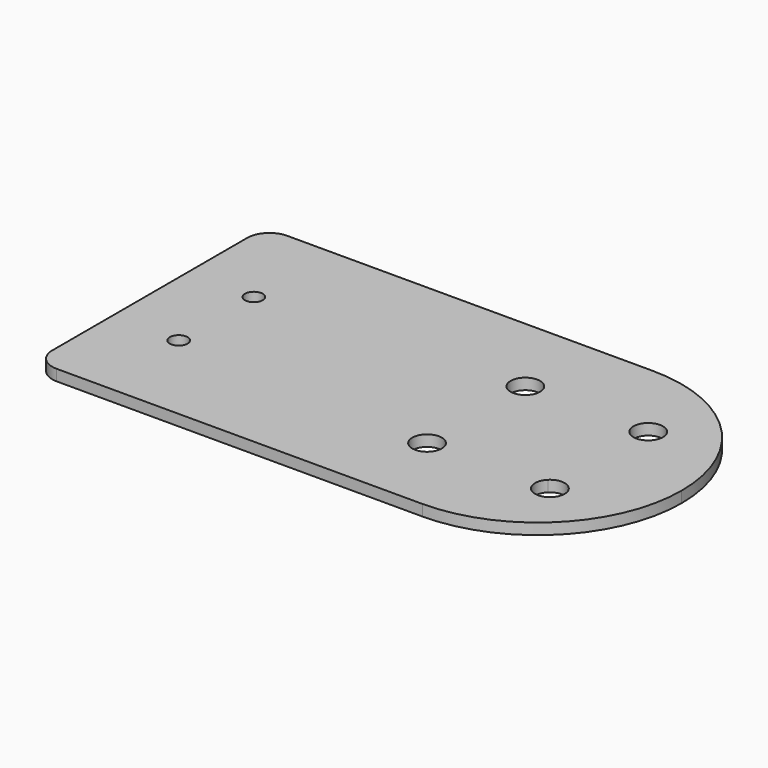
from build123d import *

# Parameters (mm, degrees)
F0_R     = 2.54
F1_DEPTH = 3.175


# Not quite as in the source:
# - a feature names something its author has since deleted; it is built from what else it names


with BuildPart() as f1:
    # F0 (on Top) → F1 (new body)
    with BuildSketch(Plane.XY):
        with BuildLine():
            ThreePointArc((-41.275, 0), (-29.1858323935, 29.1858323935), (0, 41.275))
            Line((0, 41.275), (-104.775, 41.275))
            ThreePointArc((-104.775, 41.275), (-109.2651280605, 39.4151280605), (-111.125, 34.925))
            Line((-111.125, 34.925), (-111.125, 0))
            Line((-111.125, 0), (-41.275, 0))
        make_face()
        with Locations((-92.075, 13.462)):
            Circle(F0_R, mode=Mode.SUBTRACT)
        with BuildLine():
            Line((-104.775, -41.275), (0, -41.275))
            ThreePointArc((0, -41.275), (-29.1858323935, -29.1858323935), (-41.275, 0))
            Line((-41.275, 0), (-111.125, 0))
            Line((-111.125, 0), (-111.125, -34.925))
            ThreePointArc((-111.125, -34.925), (-109.2651280605, -39.4151280605), (-104.775, -41.275))
        make_face()
        with Locations((-92.075, -13.462)):
            Circle(F0_R, mode=Mode.SUBTRACT)
        with BuildLine():
            Line((0, 2.8299858928), (0, 41.275))
            ThreePointArc((0, 41.275), (-29.1858323935, 29.1858323935), (-41.275, 0))
            Line((-41.275, 0), (0, 0))
            Line((0, 0), (0, 2.8299858928))
        make_face()
        with BuildLine():
            ThreePointArc((-13.3722019973, 17.6013019973), (-13.6941230664, 15.9828954935), (-14.610876709, 14.610876709))
            ThreePointArc((-14.610876709, 14.610876709), (-21.5084809282, 19.2197085011), (-13.3722019973, 17.6013019973))
        make_face(mode=Mode.SUBTRACT)
        with BuildLine():
            ThreePointArc((-41.275, 0), (-29.1858323935, -29.1858323935), (0, -41.275))
            Line((0, -41.275), (0, 0))
            Line((0, 0), (-41.275, 0))
        make_face()
        with BuildLine():
            ThreePointArc((-13.3722019973, -17.6013019973), (-21.5084809282, -19.2197085011), (-14.610876709, -14.610876709))
            ThreePointArc((-14.610876709, -14.610876709), (-13.6941230664, -15.9828954935), (-13.3722019973, -17.6013019973))
        make_face(mode=Mode.SUBTRACT)
        with BuildLine():
            ThreePointArc((0, -41.275), (29.1858323935, -29.1858323935), (41.275, 0))
            ThreePointArc((41.275, 0), (29.1858323935, 29.1858323935), (0, 41.275))
            Line((0, 41.275), (0, 2.8299858928))
            Line((0, 2.8299858928), (0, 0))
            Line((0, 0), (0, -41.275))
        make_face()
        with BuildLine():
            ThreePointArc((21.8304019973, -17.6013019973), (15.9828954935, -21.5084809282), (14.610876709, -14.610876709))
            ThreePointArc((14.610876709, -14.610876709), (19.2197085011, -13.6941230664), (21.8304019973, -17.6013019973))
        make_face(mode=Mode.SUBTRACT)
        with BuildLine():
            ThreePointArc((21.8304019973, 17.6013019973), (19.2197085011, 13.6941230664), (14.610876709, 14.610876709))
            ThreePointArc((14.610876709, 14.610876709), (15.9828954935, 21.5084809282), (21.8304019973, 17.6013019973))
        make_face(mode=Mode.SUBTRACT)
    extrude(amount=F1_DEPTH)


solid = f1.part
